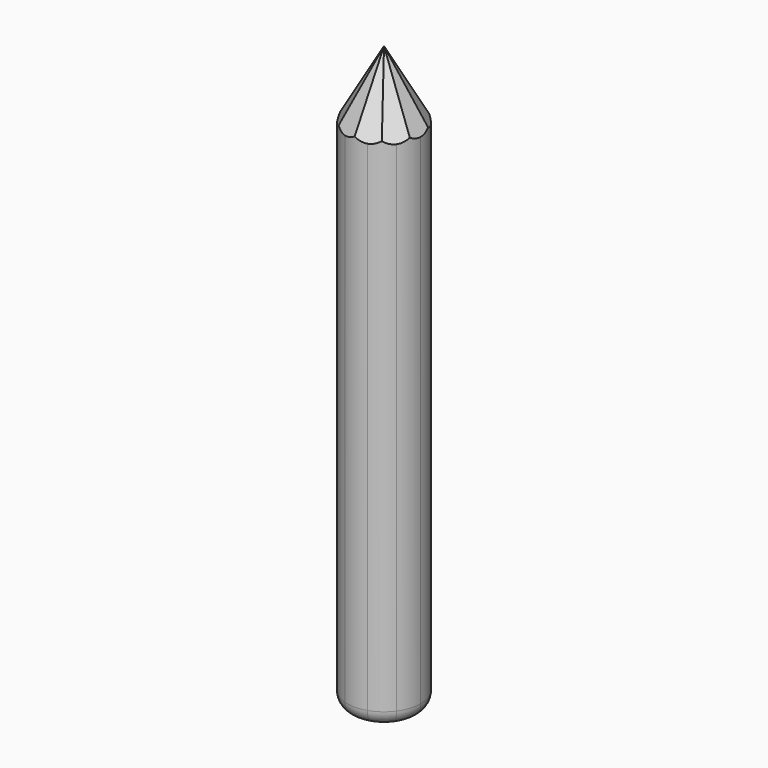
from build123d import *

# Parameters (mm, degrees)
F1_DEPTH     = 177.8
F4_R         = 12.69999
F5_T1_DEPTH  = 6.4984e-06
F5_T3_DEPTH  = 6.4984e-06
F5_T5_DEPTH  = 6.4984e-06
F5_T7_DEPTH  = 6.4984e-06
F5_T9_DEPTH  = 6.4984e-06
F5_T11_DEPTH = 6.4984e-06
F5_T13_DEPTH = 6.4984e-06
F5_T15_DEPTH = 6.4984e-06
F5_T17_DEPTH = 6.4984e-06
F5_T20_ANGLE = 36
F5_T22_ANGLE = 36
F5_T24_ANGLE = 36
F5_T26_ANGLE = 36
F5_T28_ANGLE = 36
F5_T30_ANGLE = 36
F5_T32_ANGLE = 36
F5_T34_ANGLE = 36
F5_T36_ANGLE = 36
F5_T38_ANGLE = 36


# Not quite as in the source:
# - a fillet or chamfer that OpenCascade refuses, or shapes differently, is made with other operations: its cross-section is extruded or revolved along the edge and cut away or added
# - a fillet or chamfer is up to 0.001 mm smaller than in the source, because OpenCascade refuses the exact size


with BuildPart() as f1:
    # F0 (on Top) → F1 (new body)
    with BuildSketch(Plane.XY):
        Polygon((-12.7, 4.1264801422), (-12.7, -4.1264801422), (-7.8490316571, -10.8032652661), (0, -13.3535702478), (7.8490316571, -10.8032652661), (12.7, -4.1264801422), (12.7, 4.1264801422), (7.8490316571, 10.8032652661), (0, 13.3535702478), (-7.8490316571, 10.8032652661), align=None)
    extrude(amount=F1_DEPTH)

    # F1_face (on face) → F3 section 0
    with BuildSketch(Plane.XY.offset(177.8), mode=Mode.PRIVATE) as f3_s0:
        Polygon((-7.8490316571, 10.8032652661), (-12.7, 4.1264801422), (-12.7, -4.1264801422), (-7.8490316571, -10.8032652661), (0, -13.3535702478), (7.8490316571, -10.8032652661), (12.7, -4.1264801422), (12.7, 4.1264801422), (7.8490316571, 10.8032652661), (0, 13.3535702478), align=None)
    loft([f3_s0.sketch, Vertex(0, 0, 201.3573497534)])

    # F4 (radius 12.7 in the source; OpenCascade refuses exactly that, so slightly less here)
    f4_edges = [f1.edges().sort_by_distance(p)[0] for p in [
        (0, -13.35357, 88.9),
        (-7.849032, -10.803265, 88.9),
        (-12.7, -4.12648, 88.9),
        (-12.7, 4.12648, 88.9),
        (-7.849032, 10.803265, 88.9),
        (0, 13.35357, 88.9),
        (7.849032, 10.803265, 88.9),
        (12.7, 4.12648, 88.9),
        (12.7, -4.12648, 88.9),
        (7.849032, -10.803265, 88.9),
    ]]
    fillet(f4_edges, radius=F4_R)

    # F5: fillet of radius 5.08 on 1 edges, made by hand

    # F5_s2 → F5_t1 (cut)
    with BuildSketch(Plane.XZ.offset(-3.2492e-06)):
        with BuildLine():
            ThreePointArc((-7.62, 0), (-11.2121024484, 1.4878975516), (-12.7, 5.08))
            Line((-12.7, 5.08), (-12.7, 0))
            Line((-12.7, 0), (-7.62, 0))
        make_face()
        with BuildLine():
            ThreePointArc((7.62, 0), (11.2121024484, 1.4878975516), (12.7, 5.08))
            Line((12.7, 5.08), (12.7, 0))
            Line((12.7, 0), (7.62, 0))
        make_face()
    extrude(amount=F5_T1_DEPTH, mode=Mode.SUBTRACT)

    # F5_s4 → F5_t3 (cut)
    with BuildSketch(Plane(origin=(-1.9098e-06, 2.6287e-06, 0), x_dir=(0, 0, 1), z_dir=(0.5877852523, -0.8090169944, 0))):
        with BuildLine():
            ThreePointArc((0, 7.62), (1.4878975516, 11.2121024484), (5.08, 12.7))
            Line((5.08, 12.7), (0, 12.7))
            Line((0, 12.7), (0, 7.62))
        make_face()
    extrude(amount=F5_T3_DEPTH, mode=Mode.SUBTRACT)

    # F5_s6 → F5_t5 (cut)
    with BuildSketch(Plane(origin=(-3.0902e-06, 1.0041e-06, 0), x_dir=(0, 0, 1), z_dir=(0.9510565163, -0.3090169944, 0))):
        with BuildLine():
            ThreePointArc((0, 7.62), (1.4878975516, 11.2121024484), (5.08, 12.7))
            Line((5.08, 12.7), (0, 12.7))
            Line((0, 12.7), (0, 7.62))
        make_face()
    extrude(amount=F5_T5_DEPTH, mode=Mode.SUBTRACT)

    # F5_s8 → F5_t7 (cut)
    with BuildSketch(Plane(origin=(-3.0902e-06, -1.0041e-06, 0), x_dir=(0, 0, 1), z_dir=(0.9510565163, 0.3090169944, 0))):
        with BuildLine():
            ThreePointArc((0, 7.62), (1.4878975516, 11.2121024484), (5.08, 12.7))
            Line((5.08, 12.7), (0, 12.7))
            Line((0, 12.7), (0, 7.62))
        make_face()
    extrude(amount=F5_T7_DEPTH, mode=Mode.SUBTRACT)

    # F5_s10 → F5_t9 (cut)
    with BuildSketch(Plane(origin=(-1.9098e-06, -2.6287e-06, 0), x_dir=(0, 0, 1), z_dir=(0.5877852523, 0.8090169944, 0))):
        with BuildLine():
            ThreePointArc((0, 7.62), (1.4878975516, 11.2121024484), (5.08, 12.7))
            Line((5.08, 12.7), (0, 12.7))
            Line((0, 12.7), (0, 7.62))
        make_face()
    extrude(amount=F5_T9_DEPTH, mode=Mode.SUBTRACT)

    # F5_s12 → F5_t11 (cut)
    with BuildSketch(Plane(origin=(1.9098e-06, -2.6287e-06, 0), x_dir=(0, 0, 1), z_dir=(-0.5877852523, 0.8090169944, 0))):
        with BuildLine():
            ThreePointArc((0, 7.62), (1.4878975516, 11.2121024484), (5.08, 12.7))
            Line((5.08, 12.7), (0, 12.7))
            Line((0, 12.7), (0, 7.62))
        make_face()
    extrude(amount=F5_T11_DEPTH, mode=Mode.SUBTRACT)

    # F5_s14 → F5_t13 (cut)
    with BuildSketch(Plane(origin=(3.0902e-06, -1.0041e-06, 0), x_dir=(0, 0, 1), z_dir=(-0.9510565163, 0.3090169944, 0))):
        with BuildLine():
            ThreePointArc((0, 7.62), (1.4878975516, 11.2121024484), (5.08, 12.7))
            Line((5.08, 12.7), (0, 12.7))
            Line((0, 12.7), (0, 7.62))
        make_face()
    extrude(amount=F5_T13_DEPTH, mode=Mode.SUBTRACT)

    # F5_s16 → F5_t15 (cut)
    with BuildSketch(Plane(origin=(3.0902e-06, 1.0041e-06, 0), x_dir=(0, 0, 1), z_dir=(-0.9510565163, -0.3090169944, 0))):
        with BuildLine():
            ThreePointArc((0, 7.62), (1.4878975516, 11.2121024484), (5.08, 12.7))
            Line((5.08, 12.7), (0, 12.7))
            Line((0, 12.7), (0, 7.62))
        make_face()
    extrude(amount=F5_T15_DEPTH, mode=Mode.SUBTRACT)

    # F5_s18 → F5_t17 (cut)
    with BuildSketch(Plane(origin=(1.9098e-06, 2.6287e-06, 0), x_dir=(0, 0, 1), z_dir=(-0.5877852523, -0.8090169944, 0))):
        with BuildLine():
            ThreePointArc((5.08, 12.7), (1.4878975516, 11.2121024484), (0, 7.62))
            Line((0, 7.62), (0, 12.7))
            Line((0, 12.7), (5.08, 12.7))
        make_face()
    extrude(amount=F5_T17_DEPTH, mode=Mode.SUBTRACT)

    # F5_s19 → F5_t20 (revolve, cut)
    with BuildSketch(Plane.XZ.offset(3.2492e-06)):
        with BuildLine():
            ThreePointArc((-7.62, 0), (-11.2121024484, 1.4878975516), (-12.7, 5.08))
            Line((-12.7, 5.08), (-12.7, 0))
            Line((-12.7, 0), (-7.62, 0))
        make_face()
    revolve(axis=Axis((-1e-05, -3.2492e-06, 0), (0, 0, 1)), revolution_arc=F5_T20_ANGLE, mode=Mode.SUBTRACT)

    # F5_s21 → F5_t22 (revolve, cut)
    with BuildSketch(Plane(origin=(1.9098e-06, -2.6287e-06, 0), x_dir=(0, 0, 1), z_dir=(-0.5877852523, 0.8090169944, 0))):
        with BuildLine():
            ThreePointArc((0, -7.62), (1.4878975516, -11.2121024484), (5.08, -12.7))
            Line((5.08, -12.7), (0, -12.7))
            Line((0, -12.7), (0, -7.62))
        make_face()
    revolve(axis=Axis((-6.1803e-06, -8.5065e-06, 0), (0, 0, 1)), revolution_arc=F5_T22_ANGLE, mode=Mode.SUBTRACT)

    # F5_s23 → F5_t24 (revolve, cut)
    with BuildSketch(Plane(origin=(3.0902e-06, -1.0041e-06, 0), x_dir=(0, 0, 1), z_dir=(-0.9510565163, 0.3090169944, 0))):
        with BuildLine():
            ThreePointArc((0, -7.62), (1.4878975516, -11.2121024484), (5.08, -12.7))
            Line((5.08, -12.7), (0, -12.7))
            Line((0, -12.7), (0, -7.62))
        make_face()
    revolve(axis=Axis((0, -1.05146e-05, 0), (0, 0, 1)), revolution_arc=F5_T24_ANGLE, mode=Mode.SUBTRACT)

    # F5_s25 → F5_t26 (revolve, cut)
    with BuildSketch(Plane(origin=(3.0902e-06, 1.0041e-06, 0), x_dir=(0, 0, 1), z_dir=(-0.9510565163, -0.3090169944, 0))):
        with BuildLine():
            ThreePointArc((0, -7.62), (1.4878975516, -11.2121024484), (5.08, -12.7))
            Line((5.08, -12.7), (0, -12.7))
            Line((0, -12.7), (0, -7.62))
        make_face()
    revolve(axis=Axis((6.1803e-06, -8.5065e-06, 0), (0, 0, 1)), revolution_arc=F5_T26_ANGLE, mode=Mode.SUBTRACT)

    # F5_s27 → F5_t28 (revolve, cut)
    with BuildSketch(Plane(origin=(1.9098e-06, 2.6287e-06, 0), x_dir=(0, 0, 1), z_dir=(-0.5877852523, -0.8090169944, 0))):
        with BuildLine():
            ThreePointArc((0, -7.62), (1.4878975516, -11.2121024484), (5.08, -12.7))
            Line((5.08, -12.7), (0, -12.7))
            Line((0, -12.7), (0, -7.62))
        make_face()
    revolve(axis=Axis((1e-05, -3.2492e-06, 0), (0, 0, 1)), revolution_arc=F5_T28_ANGLE, mode=Mode.SUBTRACT)

    # F5_s29 → F5_t30 (revolve, cut)
    with BuildSketch(Plane.XZ.offset(-3.2492e-06)):
        with BuildLine():
            ThreePointArc((7.62, 0), (11.2121024484, 1.4878975516), (12.7, 5.08))
            Line((12.7, 5.08), (12.7, 0))
            Line((12.7, 0), (7.62, 0))
        make_face()
    revolve(axis=Axis((1e-05, 3.2492e-06, 0), (0, 0, 1)), revolution_arc=F5_T30_ANGLE, mode=Mode.SUBTRACT)

    # F5_s31 → F5_t32 (revolve, cut)
    with BuildSketch(Plane(origin=(3.0902e-06, -1.0041e-06, 0), x_dir=(0, 0, 1), z_dir=(-0.9510565163, 0.3090169944, 0))):
        with BuildLine():
            ThreePointArc((0, 7.62), (1.4878975516, 11.2121024484), (5.08, 12.7))
            Line((5.08, 12.7), (0, 12.7))
            Line((0, 12.7), (0, 7.62))
        make_face()
    revolve(axis=Axis((6.1803e-06, 8.5065e-06, 0), (0, 0, -1)), revolution_arc=F5_T32_ANGLE, mode=Mode.SUBTRACT)

    # F5_s33 → F5_t34 (revolve, cut)
    with BuildSketch(Plane(origin=(3.0902e-06, 1.0041e-06, 0), x_dir=(0, 0, 1), z_dir=(-0.9510565163, -0.3090169944, 0))):
        with BuildLine():
            ThreePointArc((0, 7.62), (1.4878975516, 11.2121024484), (5.08, 12.7))
            Line((5.08, 12.7), (0, 12.7))
            Line((0, 12.7), (0, 7.62))
        make_face()
    revolve(axis=Axis((0, 1.05146e-05, 0), (0, 0, -1)), revolution_arc=F5_T34_ANGLE, mode=Mode.SUBTRACT)

    # F5_s35 → F5_t36 (revolve, cut)
    with BuildSketch(Plane(origin=(1.9098e-06, 2.6287e-06, 0), x_dir=(0, 0, 1), z_dir=(-0.5877852523, -0.8090169944, 0))):
        with BuildLine():
            ThreePointArc((0, 7.62), (1.4878975516, 11.2121024484), (5.08, 12.7))
            Line((5.08, 12.7), (0, 12.7))
            Line((0, 12.7), (0, 7.62))
        make_face()
    revolve(axis=Axis((-6.1803e-06, 8.5065e-06, 0), (0, 0, -1)), revolution_arc=F5_T36_ANGLE, mode=Mode.SUBTRACT)

    # F5_s37 → F5_t38 (revolve, cut)
    with BuildSketch(Plane(origin=(-1.9098e-06, -2.6287e-06, 0), x_dir=(0, 0, 1), z_dir=(0.5877852523, 0.8090169944, 0))):
        with BuildLine():
            ThreePointArc((0, -7.62), (1.4878975516, -11.2121024484), (5.08, -12.7))
            Line((5.08, -12.7), (0, -12.7))
            Line((0, -12.7), (0, -7.62))
        make_face()
    revolve(axis=Axis((-1e-05, 3.2492e-06, 0), (0, 0, 1)), revolution_arc=F5_T38_ANGLE, mode=Mode.SUBTRACT)


solid = f1.part
